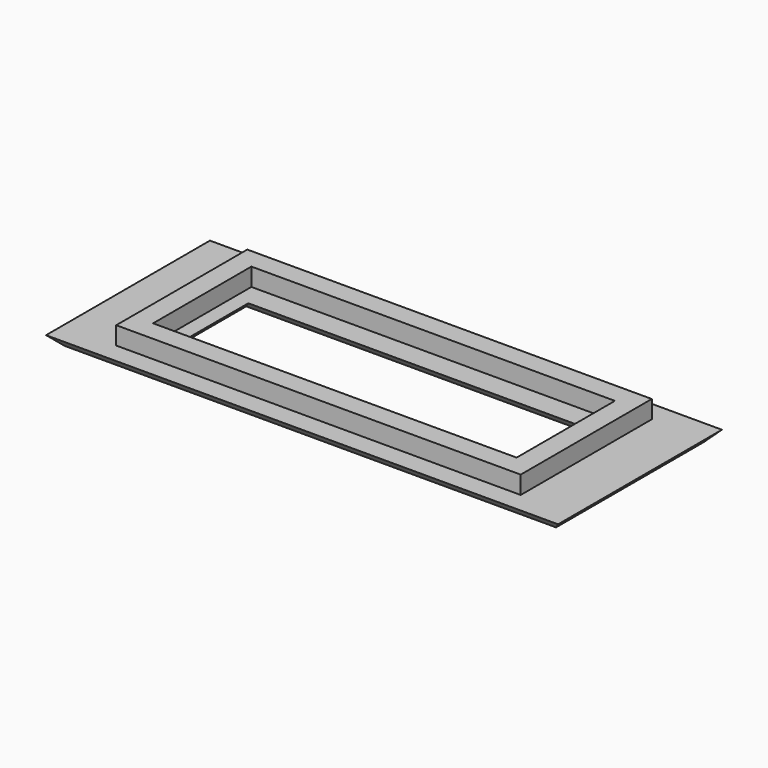
from build123d import *

# Parameters (mm, degrees)
F0_W     = 100
F0_H     = 40
F1_DEPTH = 2
F2_W     = 79
F2_H     = 32
F2_W_2   = 71
F2_H_2   = 24
F3_DEPTH = 3.5
F4_W     = 65
F4_H     = 15
F5_DEPTH = 2
F6_SIZE  = 1.99999


# Not quite as in the source:
# - a fillet or chamfer is up to 0.001 mm smaller than in the source, because OpenCascade refuses the exact size


with BuildPart() as f1:
    # F0 (on Top) → F1 (new body)
    with BuildSketch(Plane.XY):
        Rectangle(F0_W, F0_H)
    extrude(amount=F1_DEPTH)

    # F2 (on face) → F3 (join)
    with BuildSketch(Plane.XY.offset(2)):
        Rectangle(F2_W, F2_H)
        Rectangle(F2_W_2, F2_H_2, mode=Mode.SUBTRACT)
    extrude(amount=F3_DEPTH)

    # F4 (on face) → F5 (cut, through all)
    with BuildSketch(Plane.XY.offset(2)):
        Rectangle(F4_W, F4_H)
    extrude(amount=-F5_DEPTH, mode=Mode.SUBTRACT)

    # F6 (size 2 in the source; OpenCascade refuses exactly that, so slightly less here)
    f6_edges = [f1.edges().sort_by_distance(p)[0] for p in [
        (32.5, 0, 0),
        (0, 7.5, 0),
        (-32.5, 0, 0),
        (0, -7.5, 0),
        (0, 20, 0),
        (50, 0, 0),
        (0, -20, 0),
        (-50, 0, 0),
    ]]
    chamfer(f6_edges, length=F6_SIZE)


solid = f1.part
